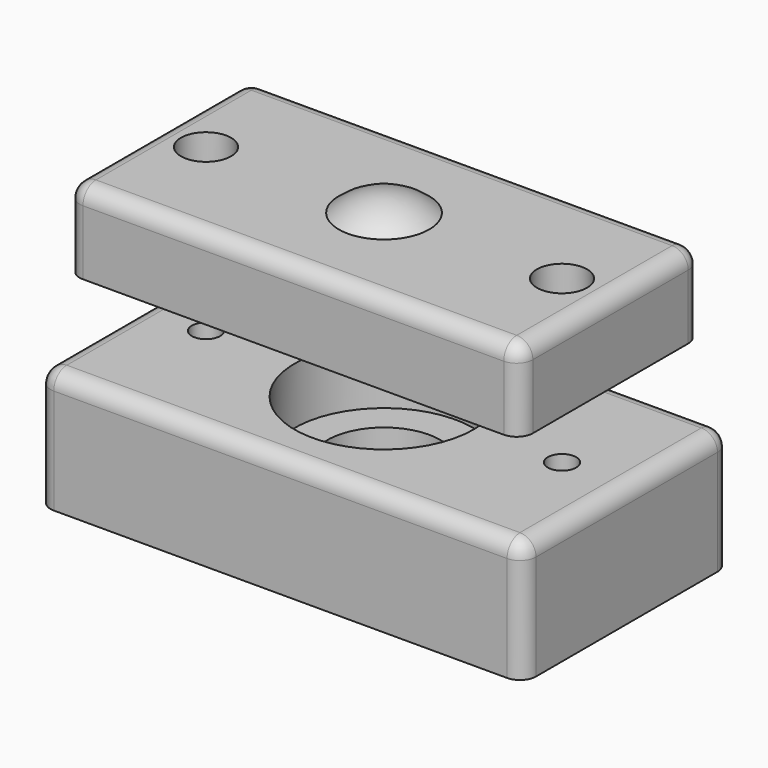
from build123d import *

# Parameters (mm, degrees)
F0_R         = 1.75
F0_R_2       = 11.05
F1_DEPTH     = 15
F0_R_3       = 7
F2_DEPTH     = 8
F4_W         = 56
F4_H         = 28
F4_R         = 1.75
F4_R_2       = 4.2
F5_DEPTH     = 10
F6_R         = 2
F7_DEPTH     = 10
F8_T1_DEPTH  = 66.0206933322
F8_T3_DEPTH  = 38.0206933322
F8_T6_ANGLE  = 90
F8_T8_ANGLE  = 90
F8_T10_ANGLE = 90
F8_T12_ANGLE = 90
F9_R         = 3.1
F9_R_2       = 1.75
F10_DEPTH    = 4


# Not quite as in the source:
# - a fillet or chamfer that OpenCascade refuses, or shapes differently, is made with other operations: its cross-section is extruded or revolved along the edge and cut away or added
# - a feature names something its author has since deleted; it is built from what else it names


with BuildPart() as f1:
    # F0 (on Top) → F1 (new body)
    with BuildSketch(Plane.XY):
        with BuildLine():
            Line((28.0103466661, 16), (-28.0103466661, 16))
            ThreePointArc((-28.0103466661, 16), (-29.4172440307, 15.4172440307), (-30, 14.0103466661))
            Line((-30, 14.0103466661), (-30, -14.0103466661))
            ThreePointArc((-30, -14.0103466661), (-29.4172440307, -15.4172440307), (-28.0103466661, -16))
            Line((-28.0103466661, -16), (28.0103466661, -16))
            ThreePointArc((28.0103466661, -16), (29.4172440307, -15.4172440307), (30, -14.0103466661))
            Line((30, -14.0103466661), (30, 14.0103466661))
            ThreePointArc((30, 14.0103466661), (29.4172440307, 15.4172440307), (28.0103466661, 16))
        make_face()
        with Locations((-22, 0)):
            Circle(F0_R, mode=Mode.SUBTRACT)
        Circle(F0_R_2, mode=Mode.SUBTRACT)
        with Locations((22, 0)):
            Circle(F0_R, mode=Mode.SUBTRACT)
    extrude(amount=F1_DEPTH)

    # F0 (on Top) → F2 (join)
    with BuildSketch(Plane.XY):
        Circle(F0_R_2)
        Circle(F0_R_3, mode=Mode.SUBTRACT)
    extrude(amount=F2_DEPTH)

    # F8: fillet of radius 2 on 8 edges, made by hand

    # F8_s2 → F8_t1 (cut)
    with BuildSketch(Plane.YZ.offset(-33.0103466661)):
        with BuildLine():
            ThreePointArc((-14, 15), (-15.4142135624, 14.4142135624), (-16, 13))
            Line((-16, 13), (-16, 15))
            Line((-16, 15), (-14, 15))
        make_face()
        with BuildLine():
            ThreePointArc((16, 13), (15.4142135624, 14.4142135624), (14, 15))
            Line((14, 15), (16, 15))
            Line((16, 15), (16, 13))
        make_face()
    extrude(amount=F8_T1_DEPTH, mode=Mode.SUBTRACT)

    # F8_s4 → F8_t3 (cut)
    with BuildSketch(Plane.XZ.offset(-19.0103466661)):
        with BuildLine():
            ThreePointArc((30, 13), (29.4142135624, 14.4142135624), (28, 15))
            Line((28, 15), (30, 15))
            Line((30, 15), (30, 13))
        make_face()
        with BuildLine():
            ThreePointArc((-28, 15), (-29.4142135624, 14.4142135624), (-30, 13))
            Line((-30, 13), (-30, 15))
            Line((-30, 15), (-28, 15))
        make_face()
    extrude(amount=F8_T3_DEPTH, mode=Mode.SUBTRACT)

    # F8_s5 → F8_t6 (revolve, cut)
    with BuildSketch(Plane.XZ.offset(-14.0103466661)):
        with BuildLine():
            ThreePointArc((30, 13), (29.4178669423, 14.4105507201), (28.0103466661, 14.9999732364))
            Line((28.0103466661, 14.9999732364), (28.0103466661, 15))
            Line((28.0103466661, 15), (30, 15))
            Line((30, 15), (30, 13))
        make_face()
    revolve(axis=Axis((28.0103466661, 14.0103466661, 15), (0, 0, 1)), revolution_arc=F8_T6_ANGLE, mode=Mode.SUBTRACT)

    # F8_s7 → F8_t8 (revolve, cut)
    with BuildSketch(Plane.YZ.offset(-28.0103466661)):
        with BuildLine():
            ThreePointArc((14.0103466661, 14.9999732364), (15.4178669423, 14.4105507201), (16, 13))
            Line((16, 13), (16, 15))
            Line((16, 15), (14.0103466661, 15))
            Line((14.0103466661, 15), (14.0103466661, 14.9999732364))
        make_face()
    revolve(axis=Axis((-28.0103466661, 14.0103466661, 15), (0, 0, 1)), revolution_arc=F8_T8_ANGLE, mode=Mode.SUBTRACT)

    # F8_s9 → F8_t10 (revolve, cut)
    with BuildSketch(Plane.XZ.offset(14.0103466661)):
        with BuildLine():
            ThreePointArc((-28.0103466661, 14.9999732364), (-29.4178669423, 14.4105507201), (-30, 13))
            Line((-30, 13), (-30, 15))
            Line((-30, 15), (-28.0103466661, 15))
            Line((-28.0103466661, 15), (-28.0103466661, 14.9999732364))
        make_face()
    revolve(axis=Axis((-28.0103466661, -14.0103466661, 15), (0, 0, 1)), revolution_arc=F8_T10_ANGLE, mode=Mode.SUBTRACT)

    # F8_s11 → F8_t12 (revolve, cut)
    with BuildSketch(Plane.YZ.offset(28.0103466661)):
        with BuildLine():
            ThreePointArc((-14.0103466661, 14.9999732364), (-15.4178669423, 14.4105507201), (-16, 13))
            Line((-16, 13), (-16, 15))
            Line((-16, 15), (-14.0103466661, 15))
            Line((-14.0103466661, 15), (-14.0103466661, 14.9999732364))
        make_face()
    revolve(axis=Axis((28.0103466661, -14.0103466661, 15), (0, 0, 1)), revolution_arc=F8_T12_ANGLE, mode=Mode.SUBTRACT)


with BuildPart() as f5:
    # F4 (on offset) → F5 (new body)
    with BuildSketch(Plane.XY.offset(25)):
        Rectangle(F4_W, F4_H)
        with Locations((-22, 0)):
            Circle(F4_R, mode=Mode.SUBTRACT)
        Circle(F4_R_2, mode=Mode.SUBTRACT)
        with Locations((22, 0)):
            Circle(F4_R, mode=Mode.SUBTRACT)
        Circle(F4_R_2)
    extrude(amount=F5_DEPTH)

    # F6
    f6_edges = [f5.edges().sort_by_distance(p)[0] for p in [
        (0, -14, 35),
        (28, 0, 35),
        (0, 14, 35),
        (-28, 0, 35),
        (-28, -14, 30),
        (-28, 14, 30),
        (28, -14, 30),
        (28, 14, 30),
    ]]
    fillet(f6_edges, radius=F6_R)

    # F4 (on offset) → F7 (cut)
    with BuildSketch(Plane.XY.offset(25)):
        Circle(F4_R_2)
    extrude(amount=F7_DEPTH, mode=Mode.SUBTRACT)

    # F9 (on face) → F10 (cut)
    with BuildSketch(Plane.XY.offset(35)):
        with Locations((-22, 0)):
            Circle(F9_R)
        with Locations((-22, 0)):
            Circle(F9_R_2, mode=Mode.SUBTRACT)
        with Locations((22, 0)):
            Circle(F9_R)
        with Locations((22, 0)):
            Circle(F9_R_2, mode=Mode.SUBTRACT)
    extrude(amount=-F10_DEPTH, mode=Mode.SUBTRACT)

    # F11 (on Front) → F12 (revolve)
    with BuildSketch(Plane.XZ):
        with BuildLine():
            Line((0, 34.9572327588), (5.6344886552, 34.9572327588))
            ThreePointArc((5.6344886552, 34.9572327588), (3.0157444319, 36.5529745163), (0, 37.1093004872))
            Line((0, 37.1093004872), (0, 34.9572327588))
        make_face()
    revolve(axis=Axis((0, 0, 36.033266623), (0, 0, -1)))


solid = Compound([f1.part, f5.part])
